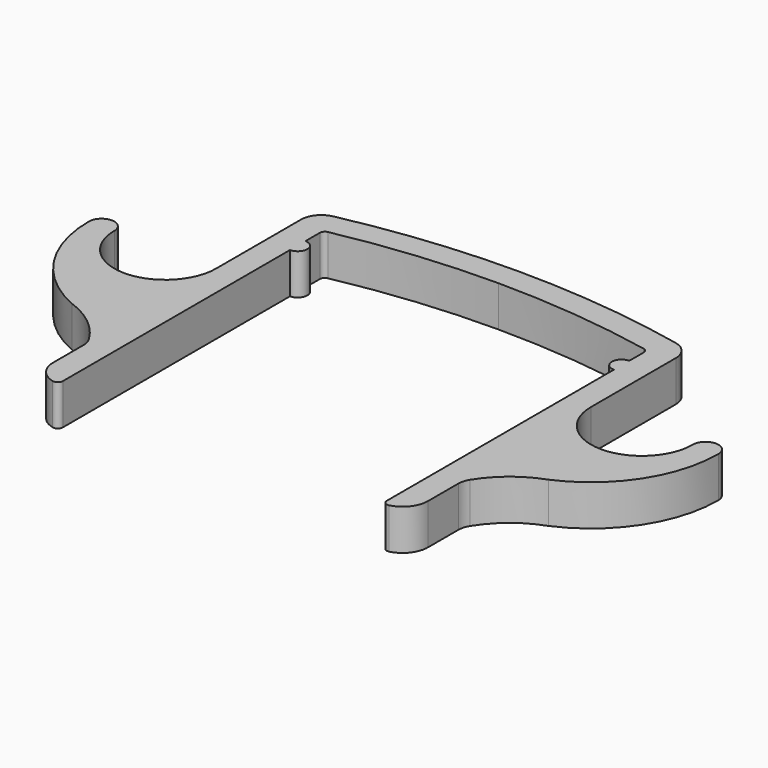
from build123d import *

# Parameters (mm, degrees)
F2_DEPTH = 10.16
F3_R     = 2.413
F4_DEPTH = 10.16
F5_R     = 5.08
F6_R     = 1.27
F8_DEPTH = 10.16
F9_R     = 5.08


# Not quite as in the source:
# - a variable given as a bare number and used for a length is read in inches; the dataset says mm whatever the document's units were
# - a feature names something its author has since deleted; it is built from what else it names


with BuildPart() as f2:
    # F1 (on Top) → F2 (new body)
    with BuildSketch(Plane.XY):
        with BuildLine():
            Line((0, 0), (0, -76.2))
            Line((0, -76.2), (0, -82.55))
            ThreePointArc((0, -82.55), (4.4901280605, -80.6901280605), (6.35, -76.2))
            Line((6.35, -76.2), (6.35, 5.1130828846))
            ThreePointArc((6.35, 5.1130828846), (-16.8661271179, 9.1115403998), (-40.386, 10.4501219109))
            ThreePointArc((-40.386, 10.4501219109), (-63.9058728821, 9.1115403998), (-87.122, 5.1130828846))
            Line((-87.122, 5.1130828846), (-87.122, -76.2))
            ThreePointArc((-87.122, -76.2), (-85.2621280605, -80.6901280605), (-80.772, -82.55))
            Line((-80.772, -82.55), (-80.772, -76.2))
            Line((-80.772, -76.2), (-80.772, 0))
            ThreePointArc((-80.772, 0), (-60.6827977504, 3.072463713), (-40.386, 4.1001219109))
            ThreePointArc((-40.386, 4.1001219109), (-20.0892022496, 3.072463713), (0, 0))
        make_face()
    extrude(amount=F2_DEPTH)

    # F3 (on Top) → F4 (join)
    with BuildSketch(Plane.XY):
        with Locations((0, -7.9375)):
            Circle(F3_R)
        with Locations((-80.772, -7.9375)):
            Circle(F3_R)
    extrude(amount=F4_DEPTH)

    # F5
    f5_edges = [f2.edges().sort_by_distance(p)[0] for p in [
        (-87.122, 5.113083, 5.08),
        (6.35, 5.113083, 5.08),
    ]]
    fillet(f5_edges, radius=F5_R)

    # F6
    f6_edges = [f2.edges().sort_by_distance(p)[0] for p in [
        (0, -82.55, 5.08),
        (-80.772, -82.55, 5.08),
        (0, 0, 5.08),
        (-80.772, 0, 5.08),
    ]]
    fillet(f6_edges, radius=F6_R)

    # F7 (on Top) → F8 (join)
    with BuildSketch(Plane.XY):
        with BuildLine():
            ThreePointArc((31.75, -25.4), (19.05, -38.1), (6.35, -25.4))
            Line((6.35, -25.4), (6.35, -65.42595876))
            ThreePointArc((6.35, -65.42595876), (11.6697145424, -58.7651555547), (19.05, -54.499355663))
            ThreePointArc((19.05, -54.499355663), (32.9139558425, -42.7901912008), (38.1, -25.4))
            ThreePointArc((38.1, -25.4), (34.925, -28.575), (31.75, -25.4))
        make_face()
        with BuildLine():
            ThreePointArc((38.1, -25.4), (34.925, -22.225), (31.75, -25.4))
            ThreePointArc((31.75, -25.4), (34.925, -28.575), (38.1, -25.4))
        make_face()
        with BuildLine():
            Line((-87.122, -65.42595876), (-87.122, -25.4))
            ThreePointArc((-87.122, -25.4), (-99.822, -38.1), (-112.522, -25.4))
            ThreePointArc((-112.522, -25.4), (-115.697, -28.575), (-118.872, -25.4))
            ThreePointArc((-118.872, -25.4), (-113.6859558425, -42.7901912008), (-99.822, -54.499355663))
            ThreePointArc((-99.822, -54.499355663), (-92.4417145424, -58.7651555547), (-87.122, -65.42595876))
        make_face()
        with BuildLine():
            ThreePointArc((-118.872, -25.4), (-115.697, -28.575), (-112.522, -25.4))
            ThreePointArc((-112.522, -25.4), (-115.697, -22.225), (-118.872, -25.4))
        make_face()
    extrude(amount=F8_DEPTH)

    # F9
    f9_edges = [f2.edges().sort_by_distance(p)[0] for p in [
        (6.35, -65.425959, 5.08),
        (-87.122, -65.425959, 5.08),
    ]]
    fillet(f9_edges, radius=F9_R)


solid = f2.part
